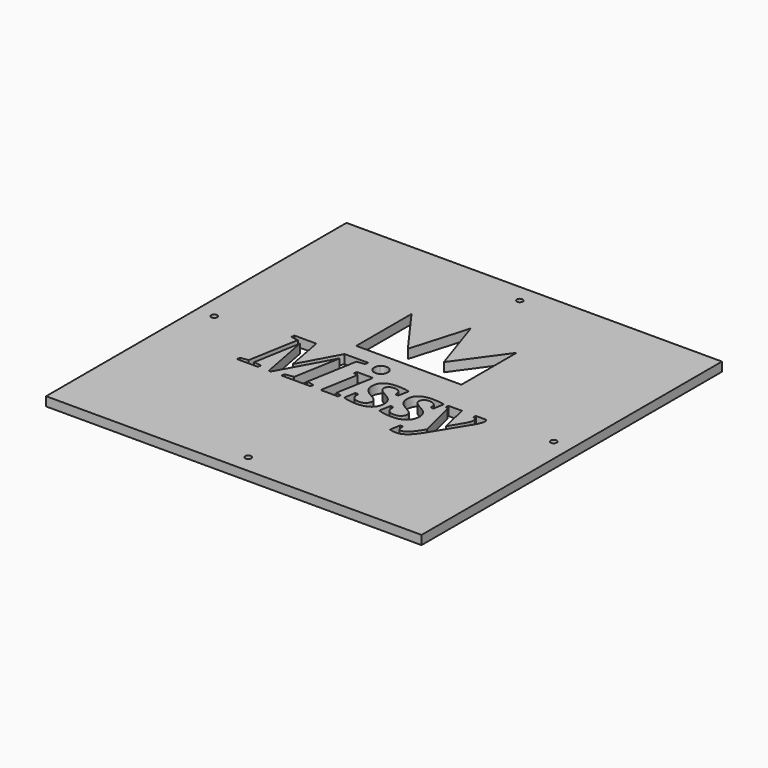
from build123d import *

# Parameters (mm, degrees)
F0_W     = 125
F0_H     = 125
F0_R     = 1
F1_DEPTH = 3


with BuildPart() as f1:
    # F0 (on Top) → F1 (new body)
    with BuildSketch(Plane.XY):
        with Locations((-316.5322542191, 138.1068900228)):
            Rectangle(F0_W, F0_H)
        Polygon((-332.7409417271, 139.9387681643), (-342.1184759568, 122.9361146688), (-342.780917002, 122.9361146688), (-346.0273479403, 139.9387681643), (-348.7710753902, 124.4066398261), (-346.2011799876, 124.0072959336), (-346.3797101984, 122.9361146688), (-353.3799737265, 122.9361146688), (-353.2061416792, 124.0072959336), (-350.6080572959, 124.4066398261), (-347.6576106545, 141.1696869861), (-350.1053538076, 141.5549363883), (-349.91742727, 142.626117653), (-342.6775574063, 142.626117653), (-340.2580032339, 129.7907351303), (-333.2671360326, 142.626117653), (-325.4118067581, 142.626117653), (-325.6044314592, 141.5549363883), (-328.2025158425, 141.1696869861), (-331.1529624839, 124.4066398261), (-328.7005211673, 124.0072959336), (-328.8790513781, 122.9361146688), (-338.5243809239, 122.9361146688), (-338.3458507131, 124.0072959336), (-335.4846691771, 124.4066398261), align=None, mode=Mode.SUBTRACT)
        Polygon((-319.0974750925, 136.7393188605), (-321.3009137466, 124.256298596), (-319.5531969463, 123.9039363378), (-319.7129345033, 122.9361146688), (-325.4822792097, 122.9361146688), (-323.283538719, 135.41443677), (-324.6178171365, 135.7667990281), (-324.4580795794, 136.7393188605), align=None, mode=Mode.SUBTRACT)
        with Locations((-316.5322542191, 81.6068900228)):
            Circle(F0_R, mode=Mode.SUBTRACT)
        with BuildLine():
            add(Edge.make_bspline(
                [(-308.0497437593, 128.926273057), (-307.7185232367, 128.2356430311), (-307.7185232367, 127.2960103427)],
                knots=[0, 0, 0, 1, 1, 1], degree=2))
            add(Edge.make_bspline(
                [(-307.7185232367, 127.2960103427), (-307.7185232367, 125.0643827079), (-309.2172373746, 123.85225654)],
                knots=[0, 0, 0, 1, 1, 1], degree=2))
            add(Edge.make_bspline(
                [(-309.2172373746, 123.85225654), (-310.7159515125, 122.640130372), (-313.6945871345, 122.640130372)],
                knots=[0, 0, 0, 1, 1, 1], degree=2))
            add(Edge.make_bspline(
                [(-313.6945871345, 122.640130372), (-314.826844524, 122.640130372), (-316.1258867156, 122.8985293613)],
                knots=[0, 0, 0, 1, 1, 1], degree=2))
            add(Edge.make_bspline(
                [(-316.1258867156, 122.8985293613), (-317.4249289072, 123.1569283506), (-318.0544828084, 123.4341199937)],
                knots=[0, 0, 0, 1, 1, 1], degree=2))
            Line((-318.0544828084, 123.4341199937), (-317.3826454363, 127.2678213621))
            Line((-317.3826454363, 127.2678213621), (-316.4101256038, 127.2678213621))
            Line((-316.4101256038, 127.2678213621), (-316.1893119221, 125.3274798607))
            add(Edge.make_bspline(
                [(-316.1893119221, 125.3274798607), (-315.2496792337, 124.0072959336), (-313.5912275388, 124.0072959336)],
                knots=[0, 0, 0, 1, 1, 1], degree=2))
            add(Edge.make_bspline(
                [(-313.5912275388, 124.0072959336), (-312.3884976977, 124.0072959336), (-311.6696786912, 124.6462461616)],
                knots=[0, 0, 0, 1, 1, 1], degree=2))
            add(Edge.make_bspline(
                [(-311.6696786912, 124.6462461616), (-310.9508596846, 125.2851963897), (-310.9508596846, 126.2389235684)],
                knots=[0, 0, 0, 1, 1, 1], degree=2))
            add(Edge.make_bspline(
                [(-310.9508596846, 126.2389235684), (-310.9508596846, 126.8120995082), (-311.3384581685, 127.2889630976)],
                knots=[0, 0, 0, 1, 1, 1], degree=2))
            add(Edge.make_bspline(
                [(-311.3384581685, 127.2889630976), (-311.7260566525, 127.7658266869), (-312.5482352548, 128.2356430311)],
                knots=[0, 0, 0, 1, 1, 1], degree=2))
            Line((-312.5482352548, 128.2356430311), (-313.5207550872, 128.7947244806))
            add(Edge.make_bspline(
                [(-313.5207550872, 128.7947244806), (-315.1510178014, 129.7061681883), (-315.8252042553, 130.6974806745)],
                knots=[0, 0, 0, 1, 1, 1], degree=2))
            add(Edge.make_bspline(
                [(-315.8252042553, 130.6974806745), (-316.4993907092, 131.6887931607), (-316.4993907092, 132.9197119824)],
                knots=[0, 0, 0, 1, 1, 1], degree=2))
            add(Edge.make_bspline(
                [(-316.4993907092, 132.9197119824), (-316.4993907092, 137.105775609), (-310.9649541749, 137.105775609)],
                knots=[0, 0, 0, 1, 1, 1], degree=2))
            add(Edge.make_bspline(
                [(-310.9649541749, 137.105775609), (-309.2313318649, 137.105775609), (-307.1171583162, 136.6359592648)],
                knots=[0, 0, 0, 1, 1, 1], degree=2))
            Line((-307.1171583162, 136.6359592648), (-307.7514103808, 133.0982421932))
            Line((-307.7514103808, 133.0982421932), (-308.7192320498, 133.0982421932))
            Line((-308.7192320498, 133.0982421932), (-308.9071585874, 134.7097122537))
            add(Edge.make_bspline(
                [(-308.9071585874, 134.7097122537), (-309.2172373746, 135.0949616559), (-309.8186022951, 135.4097386065)],
                knots=[0, 0, 0, 1, 1, 1], degree=2))
            add(Edge.make_bspline(
                [(-309.8186022951, 135.4097386065), (-310.4199672157, 135.7245155571), (-311.1716733663, 135.7245155571)],
                knots=[0, 0, 0, 1, 1, 1], degree=2))
            add(Edge.make_bspline(
                [(-311.1716733663, 135.7245155571), (-312.285138102, 135.7245155571), (-312.806634244, 135.2241611506)],
                knots=[0, 0, 0, 1, 1, 1], degree=2))
            add(Edge.make_bspline(
                [(-312.806634244, 135.2241611506), (-313.3281303861, 134.7238067441), (-313.3281303861, 133.9204207955)],
                knots=[0, 0, 0, 1, 1, 1], degree=2))
            add(Edge.make_bspline(
                [(-313.3281303861, 133.9204207955), (-313.3281303861, 133.3472448556), (-312.8958993494, 132.8468904491)],
                knots=[0, 0, 0, 1, 1, 1], degree=2))
            add(Edge.make_bspline(
                [(-312.8958993494, 132.8468904491), (-312.4636683128, 132.3465360426), (-310.9931431555, 131.5243574403)],
                knots=[0, 0, 0, 1, 1, 1], degree=2))
            add(Edge.make_bspline(
                [(-310.9931431555, 131.5243574403), (-309.5977886134, 130.7491604724), (-308.9893764477, 130.1830317777)],
                knots=[0, 0, 0, 1, 1, 1], degree=2))
            add(Edge.make_bspline(
                [(-308.9893764477, 130.1830317777), (-308.380964282, 129.6169030829), (-308.0497437593, 128.926273057)],
                knots=[0, 0, 0, 1, 1, 1], degree=2))
        make_face(mode=Mode.SUBTRACT)
        with BuildLine():
            add(Edge.make_bspline(
                [(-296.3466186261, 128.926273057), (-296.0153981034, 128.2356430311), (-296.0153981034, 127.2960103427)],
                knots=[0, 0, 0, 1, 1, 1], degree=2))
            add(Edge.make_bspline(
                [(-296.0153981034, 127.2960103427), (-296.0153981034, 125.0643827079), (-297.5141122413, 123.85225654)],
                knots=[0, 0, 0, 1, 1, 1], degree=2))
            add(Edge.make_bspline(
                [(-297.5141122413, 123.85225654), (-299.0128263792, 122.640130372), (-301.9914620013, 122.640130372)],
                knots=[0, 0, 0, 1, 1, 1], degree=2))
            add(Edge.make_bspline(
                [(-301.9914620013, 122.640130372), (-303.1237193907, 122.640130372), (-304.4227615823, 122.8985293613)],
                knots=[0, 0, 0, 1, 1, 1], degree=2))
            add(Edge.make_bspline(
                [(-304.4227615823, 122.8985293613), (-305.721803774, 123.1569283506), (-306.3513576752, 123.4341199937)],
                knots=[0, 0, 0, 1, 1, 1], degree=2))
            Line((-306.3513576752, 123.4341199937), (-305.679520303, 127.2678213621))
            Line((-305.679520303, 127.2678213621), (-304.7070004706, 127.2678213621))
            Line((-304.7070004706, 127.2678213621), (-304.4861867888, 125.3274798607))
            add(Edge.make_bspline(
                [(-304.4861867888, 125.3274798607), (-303.5465541005, 124.0072959336), (-301.8881024055, 124.0072959336)],
                knots=[0, 0, 0, 1, 1, 1], degree=2))
            add(Edge.make_bspline(
                [(-301.8881024055, 124.0072959336), (-300.6853725645, 124.0072959336), (-299.9665535579, 124.6462461616)],
                knots=[0, 0, 0, 1, 1, 1], degree=2))
            add(Edge.make_bspline(
                [(-299.9665535579, 124.6462461616), (-299.2477345513, 125.2851963897), (-299.2477345513, 126.2389235684)],
                knots=[0, 0, 0, 1, 1, 1], degree=2))
            add(Edge.make_bspline(
                [(-299.2477345513, 126.2389235684), (-299.2477345513, 126.8120995082), (-299.6353330353, 127.2889630976)],
                knots=[0, 0, 0, 1, 1, 1], degree=2))
            add(Edge.make_bspline(
                [(-299.6353330353, 127.2889630976), (-300.0229315192, 127.7658266869), (-300.8451101215, 128.2356430311)],
                knots=[0, 0, 0, 1, 1, 1], degree=2))
            Line((-300.8451101215, 128.2356430311), (-301.8176299539, 128.7947244806))
            add(Edge.make_bspline(
                [(-301.8176299539, 128.7947244806), (-303.4478926682, 129.7061681883), (-304.1220791221, 130.6974806745)],
                knots=[0, 0, 0, 1, 1, 1], degree=2))
            add(Edge.make_bspline(
                [(-304.1220791221, 130.6974806745), (-304.796265576, 131.6887931607), (-304.796265576, 132.9197119824)],
                knots=[0, 0, 0, 1, 1, 1], degree=2))
            add(Edge.make_bspline(
                [(-304.796265576, 132.9197119824), (-304.796265576, 137.105775609), (-299.2618290416, 137.105775609)],
                knots=[0, 0, 0, 1, 1, 1], degree=2))
            add(Edge.make_bspline(
                [(-299.2618290416, 137.105775609), (-297.5282067317, 137.105775609), (-295.4140331829, 136.6359592648)],
                knots=[0, 0, 0, 1, 1, 1], degree=2))
            Line((-295.4140331829, 136.6359592648), (-296.0482852475, 133.0982421932))
            Line((-296.0482852475, 133.0982421932), (-297.0161069165, 133.0982421932))
            Line((-297.0161069165, 133.0982421932), (-297.2040334542, 134.7097122537))
            add(Edge.make_bspline(
                [(-297.2040334542, 134.7097122537), (-297.5141122413, 135.0949616559), (-298.1154771619, 135.4097386065)],
                knots=[0, 0, 0, 1, 1, 1], degree=2))
            add(Edge.make_bspline(
                [(-298.1154771619, 135.4097386065), (-298.7168420824, 135.7245155571), (-299.4685482331, 135.7245155571)],
                knots=[0, 0, 0, 1, 1, 1], degree=2))
            add(Edge.make_bspline(
                [(-299.4685482331, 135.7245155571), (-300.5820129688, 135.7245155571), (-301.1035091108, 135.2241611506)],
                knots=[0, 0, 0, 1, 1, 1], degree=2))
            add(Edge.make_bspline(
                [(-301.1035091108, 135.2241611506), (-301.6250052528, 134.7238067441), (-301.6250052528, 133.9204207955)],
                knots=[0, 0, 0, 1, 1, 1], degree=2))
            add(Edge.make_bspline(
                [(-301.6250052528, 133.9204207955), (-301.6250052528, 133.3472448556), (-301.1927742162, 132.8468904491)],
                knots=[0, 0, 0, 1, 1, 1], degree=2))
            add(Edge.make_bspline(
                [(-301.1927742162, 132.8468904491), (-300.7605431795, 132.3465360426), (-299.2900180223, 131.5243574403)],
                knots=[0, 0, 0, 1, 1, 1], degree=2))
            add(Edge.make_bspline(
                [(-299.2900180223, 131.5243574403), (-297.8946634801, 130.7491604724), (-297.2862513144, 130.1830317777)],
                knots=[0, 0, 0, 1, 1, 1], degree=2))
            add(Edge.make_bspline(
                [(-297.2862513144, 130.1830317777), (-296.6778391487, 129.6169030829), (-296.3466186261, 128.926273057)],
                knots=[0, 0, 0, 1, 1, 1], degree=2))
        make_face(mode=Mode.SUBTRACT)
        with BuildLine():
            add(Edge.make_bspline(
                [(-281.4369969439, 136.7393188605), (-281.0564457051, 136.4010510927), (-281.0564457051, 135.8137806625)],
                knots=[0, 0, 0, 1, 1, 1], degree=2))
            add(Edge.make_bspline(
                [(-281.0564457051, 135.8137806625), (-281.0564457051, 134.488898572), (-282.2450810558, 132.5814442146)],
                knots=[0, 0, 0, 1, 1, 1], degree=2))
            Line((-282.2450810558, 132.5814442146), (-288.6909612978, 122.0716525956))
            add(Edge.make_bspline(
                [(-288.6909612978, 122.0716525956), (-290.1004103303, 119.7648543457), (-291.0611847542, 118.6701822638)],
                knots=[0, 0, 0, 1, 1, 1], degree=2))
            add(Edge.make_bspline(
                [(-291.0611847542, 118.6701822638), (-292.021959178, 117.5755101819), (-293.0203189094, 117.0117305689)],
                knots=[0, 0, 0, 1, 1, 1], degree=2))
            add(Edge.make_bspline(
                [(-293.0203189094, 117.0117305689), (-294.0186786407, 116.4479509559), (-295.1368415398, 116.4479509559)],
                knots=[0, 0, 0, 1, 1, 1], degree=2))
            add(Edge.make_bspline(
                [(-295.1368415398, 116.4479509559), (-295.8838495271, 116.4479509559), (-296.3325241357, 116.4996307537)],
                knots=[0, 0, 0, 1, 1, 1], degree=2))
            add(Edge.make_bspline(
                [(-296.3325241357, 116.4996307537), (-296.7811987444, 116.5513105516), (-297.500017751, 116.7251425989)],
                knots=[0, 0, 0, 1, 1, 1], degree=2))
            Line((-297.500017751, 116.7251425989), (-296.8798601767, 120.2769541608))
            Line((-296.8798601767, 120.2769541608), (-296.0013036131, 120.2769541608))
            Line((-296.0013036131, 120.2769541608), (-295.7053193163, 118.4305759283))
            add(Edge.make_bspline(
                [(-295.7053193163, 118.4305759283), (-295.3388625678, 118.0923081605), (-294.681119686, 118.0923081605)],
                knots=[0, 0, 0, 1, 1, 1], degree=2))
            add(Edge.make_bspline(
                [(-294.681119686, 118.0923081605), (-293.797864959, 118.0923081605), (-292.7548726749, 119.1047623821)],
                knots=[0, 0, 0, 1, 1, 1], degree=2))
            add(Edge.make_bspline(
                [(-292.7548726749, 119.1047623821), (-291.7118803908, 120.1172166038), (-290.0816176766, 122.8609440538)],
                knots=[0, 0, 0, 1, 1, 1], degree=2))
            Line((-290.0816176766, 122.8609440538), (-293.2246890191, 135.41443677))
            Line((-293.2246890191, 135.41443677), (-294.1220382364, 135.7667990281))
            Line((-294.1220382364, 135.7667990281), (-293.957602516, 136.7393188605))
            Line((-293.957602516, 136.7393188605), (-289.5131399001, 136.7393188605))
            Line((-289.5131399001, 136.7393188605), (-287.2815122653, 127.3570864675))
            Line((-287.2815122653, 127.3570864675), (-284.6223517573, 131.7592656123))
            add(Edge.make_bspline(
                [(-284.6223517573, 131.7592656123), (-284.2277060282, 132.4076121673), (-283.9552125486, 133.1781109717)],
                knots=[0, 0, 0, 1, 1, 1], degree=2))
            add(Edge.make_bspline(
                [(-283.9552125486, 133.1781109717), (-283.682719069, 133.9486097762), (-283.682719069, 134.40433163)],
                knots=[0, 0, 0, 1, 1, 1], degree=2))
            add(Edge.make_bspline(
                [(-283.682719069, 134.40433163), (-283.682719069, 134.7848828688), (-283.8072204002, 135.026838286)],
                knots=[0, 0, 0, 1, 1, 1], degree=2))
            add(Edge.make_bspline(
                [(-283.8072204002, 135.026838286), (-283.9317217314, 135.2687937033), (-284.1384409228, 135.430880342)],
                knots=[0, 0, 0, 1, 1, 1], degree=2))
            add(Edge.make_bspline(
                [(-284.1384409228, 135.430880342), (-284.3451601143, 135.5929669808), (-285.0029029961, 135.7808935184)],
                knots=[0, 0, 0, 1, 1, 1], degree=2))
            Line((-285.0029029961, 135.7808935184), (-284.8290709488, 136.7393188605))
            Line((-284.8290709488, 136.7393188605), (-281.4369969439, 136.7393188605))
        make_face(mode=Mode.SUBTRACT)
        with Locations((-373.0322542191, 138.1068900228)):
            Circle(F0_R, mode=Mode.SUBTRACT)
        with BuildLine():
            add(Edge.make_bspline(
                [(-321.8717406048, 139.9434663278), (-322.5318325683, 140.5965110462), (-322.5318325683, 141.5549363883)],
                knots=[0, 0, 0, 1, 1, 1], degree=2))
            add(Edge.make_bspline(
                [(-322.5318325683, 141.5549363883), (-322.5318325683, 142.5086635669), (-321.8646933596, 143.1546610402)],
                knots=[0, 0, 0, 1, 1, 1], degree=2))
            add(Edge.make_bspline(
                [(-321.8646933596, 143.1546610402), (-321.1975541509, 143.8006585134), (-320.2720159529, 143.8006585134)],
                knots=[0, 0, 0, 1, 1, 1], degree=2))
            add(Edge.make_bspline(
                [(-320.2720159529, 143.8006585134), (-319.3323832646, 143.8006585134), (-318.6793385462, 143.147613795)],
                knots=[0, 0, 0, 1, 1, 1], degree=2))
            add(Edge.make_bspline(
                [(-318.6793385462, 143.147613795), (-318.0262938278, 142.4945690766), (-318.0262938278, 141.5549363883)],
                knots=[0, 0, 0, 1, 1, 1], degree=2))
            add(Edge.make_bspline(
                [(-318.0262938278, 141.5549363883), (-318.0262938278, 140.6293981903), (-318.672291301, 139.9599098998)],
                knots=[0, 0, 0, 1, 1, 1], degree=2))
            add(Edge.make_bspline(
                [(-318.672291301, 139.9599098998), (-319.3182887742, 139.2904216094), (-320.2720159529, 139.2904216094)],
                knots=[0, 0, 0, 1, 1, 1], degree=2))
            add(Edge.make_bspline(
                [(-320.2720159529, 139.2904216094), (-321.2116486412, 139.2904216094), (-321.8717406048, 139.9434663278)],
                knots=[0, 0, 0, 1, 1, 1], degree=2))
        make_face(mode=Mode.SUBTRACT)
        Polygon((-298.7825345993, 148.1166481972), (-333.7825345993, 148.1166481972), (-333.7825345993, 171.1166481972), (-322.2760232201, 155.2082197974), (-316.6692280769, 174.3719875813), (-310.2890459785, 155.2082197974), (-298.7825345993, 171.1166481972), align=None, mode=Mode.SUBTRACT)
        with Locations((-260.0322542191, 138.1068900228)):
            Circle(F0_R, mode=Mode.SUBTRACT)
        with Locations((-316.5322542191, 194.6068900228)):
            Circle(F0_R, mode=Mode.SUBTRACT)
    extrude(amount=F1_DEPTH)


solid = f1.part
